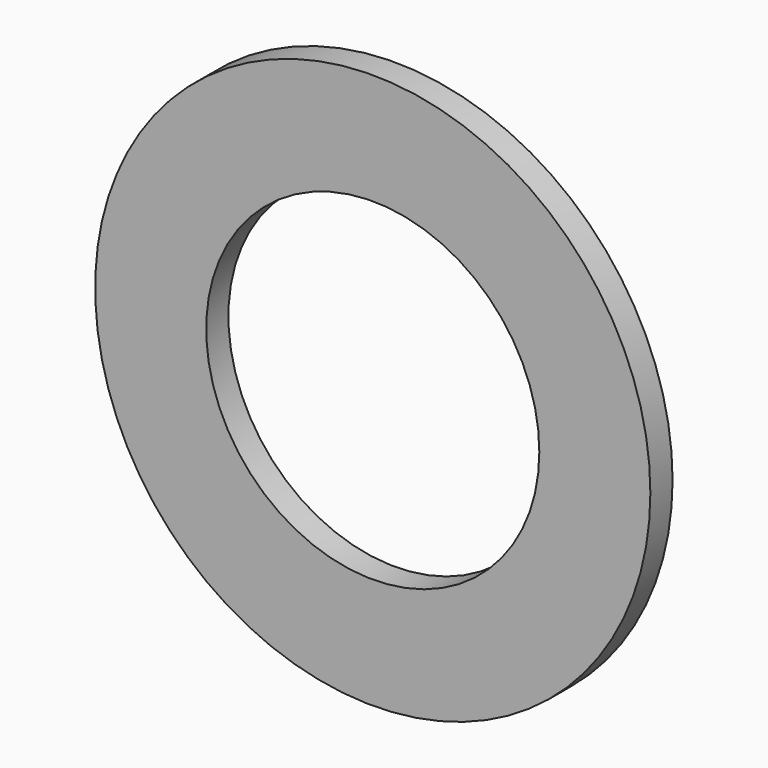
from build123d import *

# Parameters (mm, degrees)
F0_R     = 15.875
F1_DEPTH = 0.79375
F2_R     = 9.525
F3_DEPTH = 1.5885


# Not quite as in the source:
# - the program builds the solid bodies; features that only make, move or delete a surface that nothing else refers to are left out


with BuildPart() as f1:
    # F0 (on Front) → F1 (new body, symmetric)
    with BuildSketch(Plane.XZ):
        Circle(F0_R)
    extrude(amount=F1_DEPTH, both=True)

    # F2 (on face) → F3 (cut, through all)
    with BuildSketch(Plane.XZ.offset(0.79375)):
        Circle(F2_R)
    extrude(amount=-F3_DEPTH, mode=Mode.SUBTRACT)


solid = f1.part
